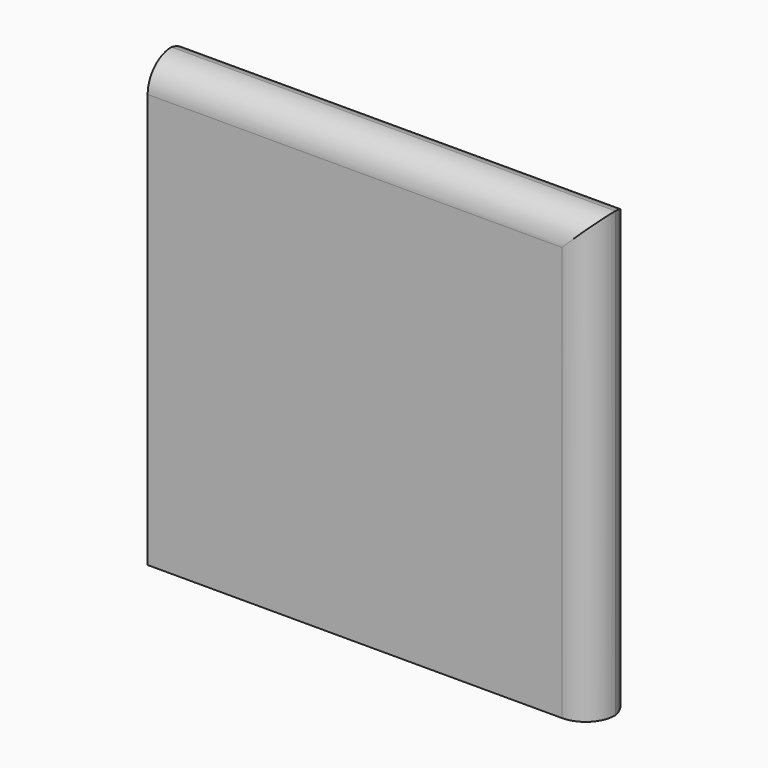
from build123d import *

# Parameters (mm, degrees)
F0_W        = 38.1
F0_H        = 38.1
F1_DEPTH    = 4.699
F2_R        = 2.54
F3_T1_DEPTH = 50.6563121576
F4_T1_DEPTH = 48.26
F5_T1_DEPTH = 48.1450497261


# Not quite as in the source:
# - a fillet or chamfer that OpenCascade refuses, or shapes differently, is made with other operations: its cross-section is extruded or revolved along the edge and cut away or added


with BuildPart() as f1:
    # F0 (on Front) → F1 (new body)
    with BuildSketch(Plane.XZ):
        Rectangle(F0_W, F0_H)
    extrude(amount=F1_DEPTH)

    # F2
    f2_edges = [f1.edges().sort_by_distance(p)[0] for p in [
        (19.05, -4.699, 0),
    ]]
    fillet(f2_edges, radius=F2_R)

    # F3: fillet of radius 2.54 on 1 edges, made by hand

    # F3_s2 → F3_t1 (cut)
    with BuildSketch(Plane.XY.offset(-25.3281560788)):
        with BuildLine():
            ThreePointArc((19.05, -2.159), (18.1946149794, -0.6139496372), (16.5387375685, 0))
            Line((16.5387375685, 0), (19.05, 0))
            Line((19.05, 0), (19.05, -2.159))
        make_face()
    extrude(amount=F3_T1_DEPTH, mode=Mode.SUBTRACT)

    # F4: fillet of radius 2.54 on 1 edges, made by hand

    # F4_s2 → F4_t1 (cut)
    with BuildSketch(Plane.YZ.offset(-25.4)):
        with BuildLine():
            ThreePointArc((-2.159, 19.05), (-3.9550512242, 18.3060512242), (-4.699, 16.51))
            Line((-4.699, 16.51), (-4.699, 19.05))
            Line((-4.699, 19.05), (-2.159, 19.05))
        make_face()
    extrude(amount=F4_T1_DEPTH, mode=Mode.SUBTRACT)

    # F5: fillet of radius 2.54 on 1 edges, made by hand

    # F5_s2 → F5_t1 (cut)
    with BuildSketch(Plane.YZ.offset(-25.3281560788)):
        with BuildLine():
            ThreePointArc((-2.159, 19.05), (-0.6139496372, 18.1946149794), (0, 16.5387375685))
            Line((0, 16.5387375685), (0, 19.05))
            Line((0, 19.05), (-2.159, 19.05))
        make_face()
    extrude(amount=F5_T1_DEPTH, mode=Mode.SUBTRACT)


solid = f1.part
